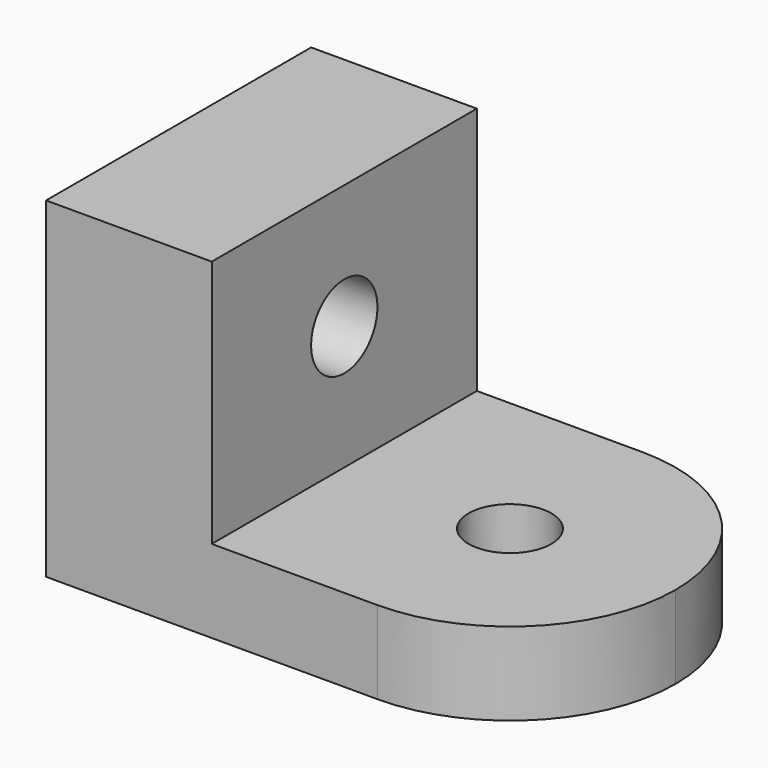
from build123d import *

# Parameters (mm, degrees)
F1_DEPTH = 40
F2_R     = 19.99999
F3_R     = 5
F4_DEPTH = 25
F5_R     = 5
F6_DEPTH = 25


# Not quite as in the source:
# - a fillet or chamfer is up to 0.001 mm smaller than in the source, because OpenCascade refuses the exact size


with BuildPart() as f1:
    # F0 (on Front) → F1 (new body)
    with BuildSketch(Plane.XZ):
        Polygon((0, -10), (0, 0), (0, 20), (-20, 20), (-20, -20), (0, -20), (40, -20), (40, -10), align=None)
    extrude(amount=F1_DEPTH)

    # F2 (radius 20 in the source; OpenCascade refuses exactly that, so slightly less here)
    f2_edges = [f1.edges().sort_by_distance(p)[0] for p in [
        (40, -40, -15),
        (40, 0, -15),
    ]]
    fillet(f2_edges, radius=F2_R)

    # F3 (on face) → F4 (cut)
    with BuildSketch(Plane.XY.offset(-10)):
        with Locations((20, -20)):
            Circle(F3_R)
    extrude(amount=-F4_DEPTH, mode=Mode.SUBTRACT)

    # F5 (on face) → F6 (cut)
    with BuildSketch(Plane.YZ):
        with Locations((-20, 5)):
            Circle(F5_R)
    extrude(amount=-F6_DEPTH, mode=Mode.SUBTRACT)


solid = f1.part
